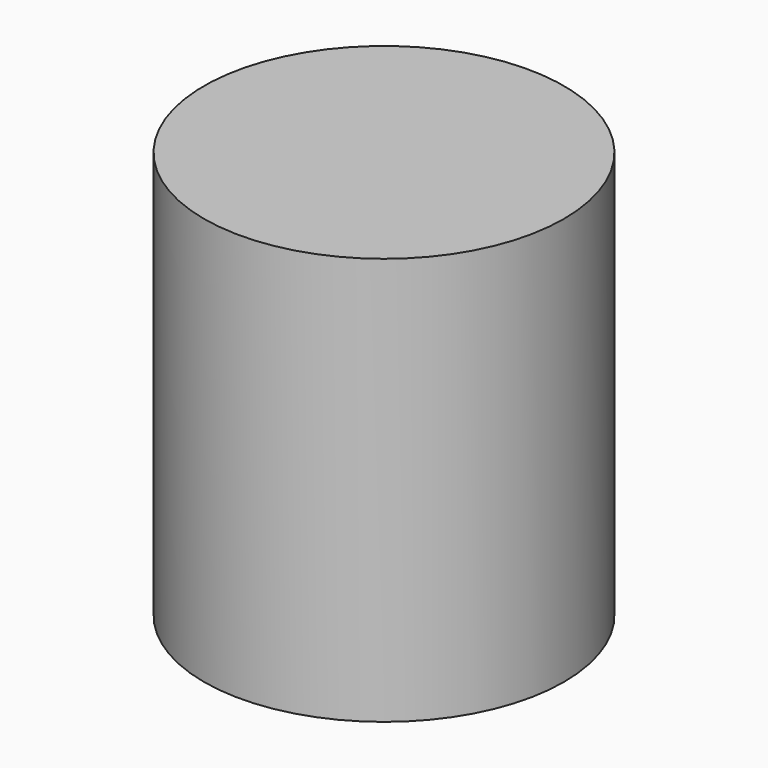
from build123d import *

# Parameters (mm, degrees)
F0_R     = 33.6408232846
F1_DEPTH = 76.2


# Not quite as in the source:
# - the program builds the solid bodies; features that only make, move or delete a surface that nothing else refers to are left out


with BuildPart() as f1:
    # F0 (on Top) → F1 (new body)
    with BuildSketch(Plane.XY):
        Circle(F0_R)
    extrude(amount=F1_DEPTH)


solid = f1.part
